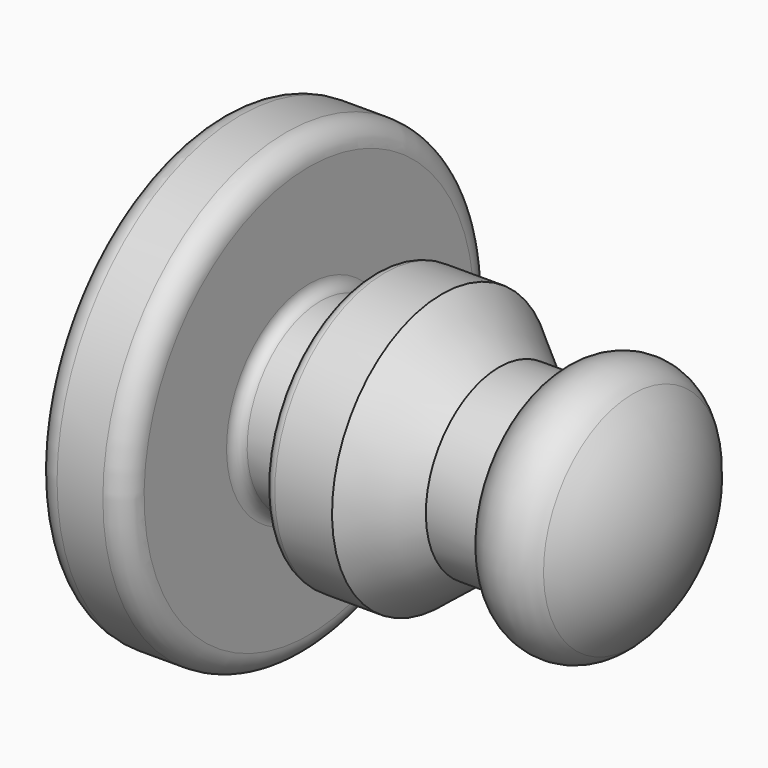
from build123d import *

# Parameters (mm, degrees)
F2_R = 0.635
F3_R = 0.635
F4_R = 0.3175
F5_R = 0.3175


# Not quite as in the source:
# - a fillet or chamfer that OpenCascade refuses, or shapes differently, is made with other operations: its cross-section is extruded or revolved along the edge and cut away or added


with BuildPart() as f1:
    # F0 (on Front) → F1 (revolve)
    with BuildSketch(Plane.XZ):
        with BuildLine():
            Line((-12.7, 0), (0, 0))
            ThreePointArc((0, 0), (-0.9357326302, 2.7871609809), (-3.3637836337, 4.445))
            Line((-3.3637836337, 4.445), (-3.3637836337, 2.54))
            Line((-3.3637836337, 2.54), (-4.8877836337, 2.54))
            Line((-4.8877836337, 2.54), (-6.477, 3.8062603766))
            Line((-6.477, 3.8062603766), (-8.382, 3.8062603766))
            Line((-8.382, 3.8062603766), (-8.382, 2.54))
            Line((-8.382, 2.54), (-10.16, 2.54))
            Line((-10.16, 2.54), (-10.16, 6.35))
            Line((-10.16, 6.35), (-12.7, 6.35))
            Line((-12.7, 6.35), (-12.7, 0))
        make_face()
    revolve(axis=Axis((-6.35, 0, 0), (-1, 0, 0)))

    # F2
    f2_edges = [f1.edges().sort_by_distance(p)[0] for p in [
        (-12.7, 0, -6.35),
    ]]
    fillet(f2_edges, radius=F2_R)

    # F3
    f3_edges = [f1.edges().sort_by_distance(p)[0] for p in [
        (-10.16, 0, -6.35),
    ]]
    fillet(f3_edges, radius=F3_R)

    # F4
    f4_edges = [f1.edges().sort_by_distance(p)[0] for p in [
        (-8.382, 0, -3.80626),
    ]]
    fillet(f4_edges, radius=F4_R)

    # F5
    f5_edges = [f1.edges().sort_by_distance(p)[0] for p in [
        (-10.16, 0, -2.54),
    ]]
    fillet(f5_edges, radius=F5_R)

    # F6: fillet of radius 1.27 on 2 edges, made by hand

    # F6_s1 → F6_t2 (revolve, cut)
    with BuildSketch(Plane.XZ):
        with BuildLine():
            ThreePointArc((-3.3637836337, 2.54), (-2.4405099474, 3.4716029629), (-1.1856937405, 3.0898246668))
            ThreePointArc((-1.1856937405, 3.0898246668), (-2.1787682731, 3.9216596724), (-3.3637836337, 4.445))
            Line((-3.3637836337, 4.445), (-3.3637836337, 2.54))
        make_face()
    revolve(axis=Axis((-3.3637836337, 0, 0), (-1, 0, 0)), mode=Mode.SUBTRACT)


solid = f1.part
